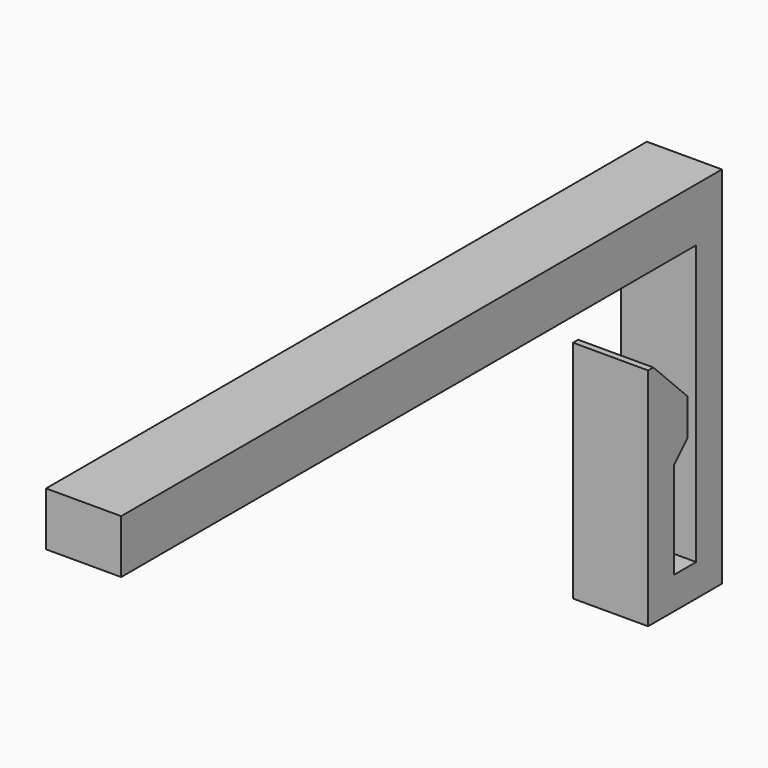
from build123d import *

# Parameters (mm, degrees)
F0_W     = 7
F0_H     = 70
F1_DEPTH = 5
F2_W     = 7
F2_H     = 3
F3_DEPTH = 26
F4_W     = 7
F4_H     = 8.6
F5_DEPTH = 3
F6_W     = 7
F6_H     = 3
F7_DEPTH = 18
F8_W     = 7
F8_H     = 9
F9_DEPTH = 1.6
F10_SIZE = 4
F11_SIZE = 1.59999


# Not quite as in the source:
# - a fillet or chamfer is up to 0.001 mm smaller than in the source, because OpenCascade refuses the exact size


with BuildPart() as f1:
    # F0 (on Top) → F1 (new body)
    with BuildSketch(Plane.XY):
        Rectangle(F0_W, F0_H)
    extrude(amount=F1_DEPTH)

    # F2 (on face) → F3 (join)
    with BuildSketch(Plane(origin=(0, 0, 0), x_dir=(1, 0, 0), z_dir=(0, 0, -1))):
        with Locations((0, -33.5)):
            Rectangle(F2_W, F2_H)
    extrude(amount=F3_DEPTH)

    # F4 (on face) → F5 (join)
    with BuildSketch(Plane(origin=(0, 0, -26), x_dir=(1, 0, 0), z_dir=(0, 0, -1))):
        with Locations((0, -30.7)):
            Rectangle(F4_W, F4_H)
    extrude(amount=F5_DEPTH)

    # F6 (on face) → F7 (join)
    with BuildSketch(Plane.XY.offset(-26)):
        with Locations((0, 27.9)):
            Rectangle(F6_W, F6_H)
    extrude(amount=F7_DEPTH)

    # F8 (on face) → F9 (join)
    with BuildSketch(Plane(origin=(0, 29.4, 0), x_dir=(-1, 0, 0), z_dir=(0, 1, 0))):
        with Locations((0, -12.5)):
            Rectangle(F8_W, F8_H)
    extrude(amount=F9_DEPTH)

    # F10
    f10_edges = [f1.edges().sort_by_distance(p)[0] for p in [
        (0, 31, -8),
    ]]
    chamfer(f10_edges, length=F10_SIZE)

    # F11 (size 1.6 in the source; OpenCascade refuses exactly that, so slightly less here)
    f11_edges = [f1.edges().sort_by_distance(p)[0] for p in [
        (0, 31, -17),
    ]]
    chamfer(f11_edges, length=F11_SIZE)


solid = f1.part
